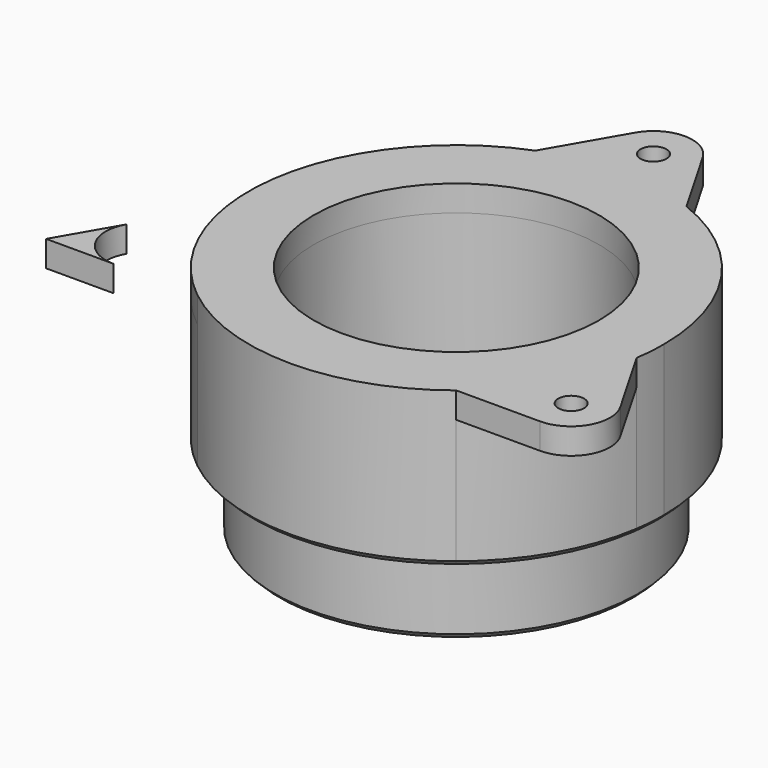
from build123d import *

# Parameters (mm, degrees)
F0_R     = 27.5
F0_R_2   = 2.5
F1_DEPTH = 5
F2_DEPTH = 25
F3_R     = 35
F3_R_2   = 27.5
F4_DEPTH = 15
F5_SIZE  = 2
F6_SIZE  = 1


with BuildPart() as f1:
    # F0 (on Top) → F1 (new body)
    with BuildSketch(Plane.XY):
        with BuildLine():
            ThreePointArc((39.5476590904, -5.998554865), (39.8867544657, -3.0077929104), (40, 0))
            ThreePointArc((40, 0), (33.0390461866, 22.5482023026), (14.5789286461, 37.248554865))
            ThreePointArc((14.5789286461, 37.248554865), (0, 40), (-14.5789286461, 37.248554865))
            ThreePointArc((-14.5789286461, 37.248554865), (-34.6410161514, 20), (-39.5476590904, -5.998554865))
            ThreePointArc((-39.5476590904, -5.998554865), (-34.6410161514, -20), (-24.9687304443, -31.25))
            ThreePointArc((-24.9687304443, -31.25), (0, -40), (24.9687304443, -31.25))
            ThreePointArc((24.9687304443, -31.25), (34.6410161514, -20), (39.5476590904, -5.998554865))
        make_face()
        Circle(F0_R, mode=Mode.SUBTRACT)
        with BuildLine():
            ThreePointArc((-14.5789286461, 37.248554865), (0, 40), (14.5789286461, 37.248554865))
            Line((14.5789286461, 37.248554865), (6.4951905284, 51.25))
            ThreePointArc((6.4951905284, 51.25), (0, 55), (-6.4951905284, 51.25))
            Line((-6.4951905284, 51.25), (-14.5789286461, 37.248554865))
        make_face()
        with Locations((0, 47.5)):
            Circle(F0_R_2, mode=Mode.SUBTRACT)
        with BuildLine():
            Line((47.6313972081, -20), (39.5476590904, -5.998554865))
            ThreePointArc((39.5476590904, -5.998554865), (34.6410161514, -20), (24.9687304443, -31.25))
            Line((24.9687304443, -31.25), (41.1362066798, -31.25))
            ThreePointArc((41.1362066798, -31.25), (47.6313972081, -27.5), (47.6313972081, -20))
        make_face()
        with Locations((41.1362066798, -23.75)):
            Circle(F0_R_2, mode=Mode.SUBTRACT)
    extrude(amount=F1_DEPTH)

    # F0 (on Top) → F2 (join)
    with BuildSketch(Plane.XY):
        with BuildLine():
            ThreePointArc((39.5476590904, -5.998554865), (39.8867544657, -3.0077929104), (40, 0))
            ThreePointArc((40, 0), (33.0390461866, 22.5482023026), (14.5789286461, 37.248554865))
            ThreePointArc((14.5789286461, 37.248554865), (0, 40), (-14.5789286461, 37.248554865))
            ThreePointArc((-14.5789286461, 37.248554865), (-34.6410161514, 20), (-39.5476590904, -5.998554865))
            ThreePointArc((-39.5476590904, -5.998554865), (-34.6410161514, -20), (-24.9687304443, -31.25))
            ThreePointArc((-24.9687304443, -31.25), (0, -40), (24.9687304443, -31.25))
            ThreePointArc((24.9687304443, -31.25), (34.6410161514, -20), (39.5476590904, -5.998554865))
        make_face()
        Circle(F0_R, mode=Mode.SUBTRACT)
    extrude(amount=-F2_DEPTH)

    # F3 (on face) → F4 (join)
    with BuildSketch(Plane(origin=(0, 0, -25), x_dir=(1, 0, 0), z_dir=(0, 0, -1))):
        Circle(F3_R)
        Circle(F3_R_2, mode=Mode.SUBTRACT)
    extrude(amount=F4_DEPTH)

    # F5
    f5_edges = [f1.edges().sort_by_distance(p)[0] for p in [
        (-2.5, 47.5, 0),
        (38.636207, -23.75, 0),
    ]]
    chamfer(f5_edges, length=F5_SIZE)

    # F6
    f6_edges = [f1.edges().sort_by_distance(p)[0] for p in [
        (39.547659, 5.998555, -25),
        (-35, 0, -40),
        (-27.5, 0, -40),
    ]]
    chamfer(f6_edges, length=F6_SIZE)


with BuildPart() as f1b:
    # F0 (on Top) → F1, piece 2 (new body)
    with BuildSketch(Plane.XY):
        with BuildLine():
            ThreePointArc((-41.1362066798, -31.25), (-47.6313972081, -27.5), (-47.6313972081, -20))
            Line((-47.6313972081, -20), (-54.1265877365, -31.25))
            Line((-54.1265877365, -31.25), (-41.1362066798, -31.25))
        make_face()
    extrude(amount=F1_DEPTH)


solid = Compound([f1.part, f1b.part])
